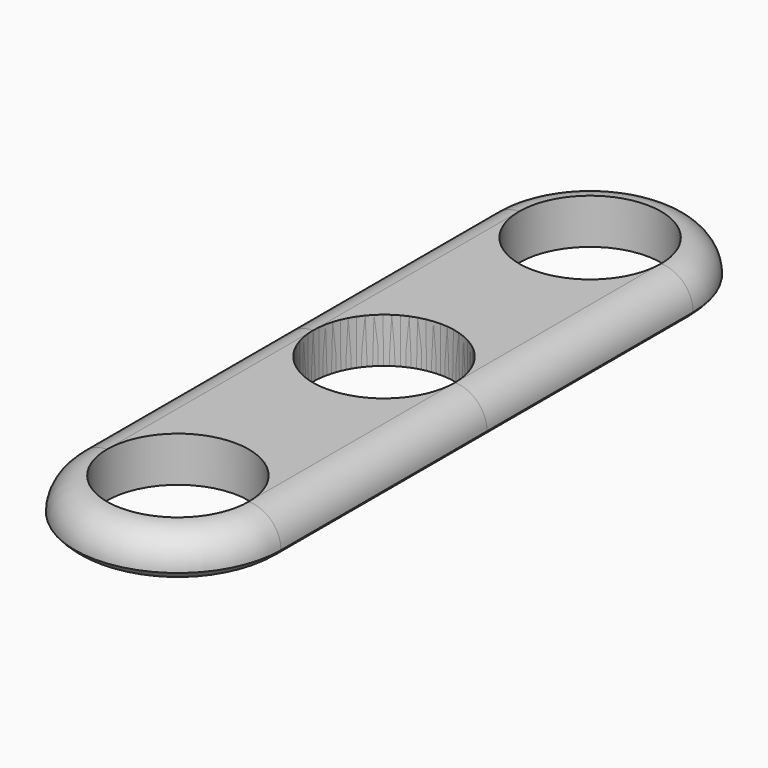
from build123d import *

# Parameters (mm, degrees)
F1_DEPTH      = 7
F2_R          = 11
F3_DEPTH      = 7
F5_COUNT      = 2
F6_R          = 4.99999
F6_2_R        = 4.99999
F7_T1_DEPTH   = 40
F7_T4_ANGLE   = 180
F7_T6_ANGLE   = 180
F7_2_T1_DEPTH = 40
F7_2_T4_ANGLE = 180
F7_2_T6_ANGLE = 180


# Not quite as in the source:
# - a fillet or chamfer that OpenCascade refuses, or shapes differently, is made with other operations: its cross-section is extruded or revolved along the edge and cut away or added
# - a fillet or chamfer is up to 0.001 mm smaller than in the source, because OpenCascade refuses the exact size


with BuildPart() as f1:
    # F0 (on Top) → F1 (new body)
    with BuildSketch(Plane.XY):
        with BuildLine():
            ThreePointArc((-16, 0), (0, -16), (16, 0))
            ThreePointArc((16, 0), (0, 16), (-16, 0))
        make_face()
        with BuildLine():
            Line((16, -40), (16, 0))
            ThreePointArc((16, 0), (0, -16), (-16, 0))
            Line((-16, 0), (-16, -40))
            ThreePointArc((-16, -40), (0, -24), (16, -40))
        make_face()
        with BuildLine():
            ThreePointArc((-16, -40), (0, -56), (16, -40))
            ThreePointArc((16, -40), (0, -24), (-16, -40))
        make_face()
    extrude(amount=F1_DEPTH)

    # F2 (on face) → F3 (cut, through all)
    with BuildSketch(Plane.XY.offset(7)):
        Circle(F2_R)
        with Locations((0, -40)):
            Circle(F2_R)
    extrude(amount=-F3_DEPTH, mode=Mode.SUBTRACT)


with BuildPart() as f5_1:
    # F5: instance of F1
    add(f1.part.rotate(Axis((0, 0, -3.6183325574), (0, 0, -1)), 1 * 360 / F5_COUNT))

    # F6#2 (radius 5 in the source; OpenCascade refuses exactly that, so slightly less here)
    f6_2_edges = [f5_1.edges().sort_by_distance(p)[0] for p in [
        (-16, 20, 7),
    ]]
    fillet(f6_2_edges, radius=F6_2_R)

    # F7#2: fillet of radius 5 on 1 edges, made by hand

    # F7_2_s2 → F7_2_t1 (cut)
    with BuildSketch(Plane.XZ.offset(-40)):
        with BuildLine():
            ThreePointArc((-16, 2.00001), (-14.2360660677, 0.5278668401), (-11.9999925, 0))
            Line((-11.9999925, 0), (-16, 0))
            Line((-16, 0), (-16, 2.00001))
        make_face()
        with BuildLine():
            ThreePointArc((11.9999925, 0), (14.2360660677, 0.5278668401), (16, 2.00001))
            Line((16, 2.00001), (16, 0))
            Line((16, 0), (11.9999925, 0))
        make_face()
    extrude(amount=F7_2_T1_DEPTH, mode=Mode.SUBTRACT)

    # F7_2_s3 → F7_2_t4 (revolve, cut)
    with BuildSketch(Plane.XZ.offset(-40)):
        with BuildLine():
            ThreePointArc((11.9999925, 0), (14.2360660677, 0.5278668401), (16, 2.00001))
            Line((16, 2.00001), (16, 0))
            Line((16, 0), (11.9999925, 0))
        make_face()
    revolve(axis=Axis((0, 40, 0), (0, 0, 1)), revolution_arc=F7_2_T4_ANGLE, mode=Mode.SUBTRACT)

    # F7_2_s5 → F7_2_t6 (revolve, cut)
    with BuildSketch(Plane.XZ):
        with BuildLine():
            ThreePointArc((-16, 2.00001), (-14.2360660677, 0.5278668401), (-11.9999925, 0))
            Line((-11.9999925, 0), (-16, 0))
            Line((-16, 0), (-16, 2.00001))
        make_face()
    revolve(axis=Axis((0, 0, 0), (0, 0, 1)), revolution_arc=F7_2_T6_ANGLE, mode=Mode.SUBTRACT)


with BuildPart() as f1_1:
    add(f1.part)

    # F6 (radius 5 in the source; OpenCascade refuses exactly that, so slightly less here)
    f6_edges = [f1_1.edges().sort_by_distance(p)[0] for p in [
        (-16, -20, 7),
    ]]
    fillet(f6_edges, radius=F6_R)

    # F7: fillet of radius 5 on 1 edges, made by hand

    # F7_s2 → F7_t1 (cut)
    with BuildSketch(Plane.XZ):
        with BuildLine():
            ThreePointArc((-11.9999925, 0), (-14.2360660677, 0.5278668401), (-16, 2.00001))
            Line((-16, 2.00001), (-16, 0))
            Line((-16, 0), (-11.9999925, 0))
        make_face()
        with BuildLine():
            ThreePointArc((16, 2.00001), (14.2360660677, 0.5278668401), (11.9999925, 0))
            Line((11.9999925, 0), (16, 0))
            Line((16, 0), (16, 2.00001))
        make_face()
    extrude(amount=F7_T1_DEPTH, mode=Mode.SUBTRACT)

    # F7_s3 → F7_t4 (revolve, cut)
    with BuildSketch(Plane.XZ):
        with BuildLine():
            ThreePointArc((16, 2.00001), (14.2360660677, 0.5278668401), (11.9999925, 0))
            Line((11.9999925, 0), (16, 0))
            Line((16, 0), (16, 2.00001))
        make_face()
    revolve(axis=Axis((0, 0, 0), (0, 0, 1)), revolution_arc=F7_T4_ANGLE, mode=Mode.SUBTRACT)

    # F7_s5 → F7_t6 (revolve, cut)
    with BuildSketch(Plane.XZ.offset(40)):
        with BuildLine():
            ThreePointArc((-11.9999925, 0), (-14.2360660677, 0.5278668401), (-16, 2.00001))
            Line((-16, 2.00001), (-16, 0))
            Line((-16, 0), (-11.9999925, 0))
        make_face()
    revolve(axis=Axis((0, -40, 0), (0, 0, 1)), revolution_arc=F7_T6_ANGLE, mode=Mode.SUBTRACT)


solid = Compound([f5_1.part, f1_1.part])
